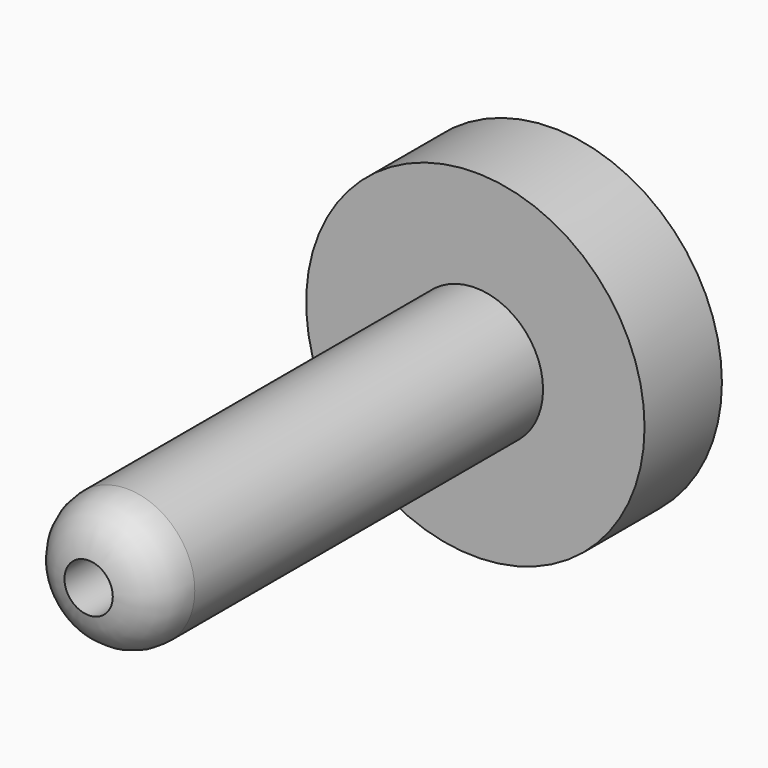
from build123d import *

# Parameters (mm, degrees)
F0_R     = 3.5
F1_DEPTH = 2
F2_R     = 1.4
F3_DEPTH = 10
F4_R     = 0.5
F5_DEPTH = 12.001


# Not quite as in the source:
# - a fillet or chamfer that OpenCascade refuses, or shapes differently, is made with other operations: its cross-section is extruded or revolved along the edge and cut away or added


with BuildPart() as f1:
    # F0 (on Front) → F1 (new body)
    with BuildSketch(Plane.XZ):
        Circle(F0_R)
    extrude(amount=F1_DEPTH)

    # F2 (on face) → F3 (join)
    with BuildSketch(Plane.XZ.offset(2)):
        Circle(F2_R)
    extrude(amount=F3_DEPTH)

    # F4 (on face) → F5 (cut, through all)
    with BuildSketch(Plane(origin=(0, 0, 0), x_dir=(-1, 0, 0), z_dir=(0, 1, 0))):
        Circle(F4_R)
    extrude(amount=-F5_DEPTH, mode=Mode.SUBTRACT)

    # F6: fillet of radius 1 on 1 edges, made by hand

    # F6_s1 → F6_t2 (revolve, cut)
    with BuildSketch(Plane.XY):
        with BuildLine():
            ThreePointArc((1.4, -11.0050125629), (1.1416198487, -11.6758329561), (0.5, -12))
            Line((0.5, -12), (1.4, -12))
            Line((1.4, -12), (1.4, -11.0050125629))
        make_face()
    revolve(axis=Axis((0, -12, 0), (0, -1, 0)), mode=Mode.SUBTRACT)


solid = f1.part
